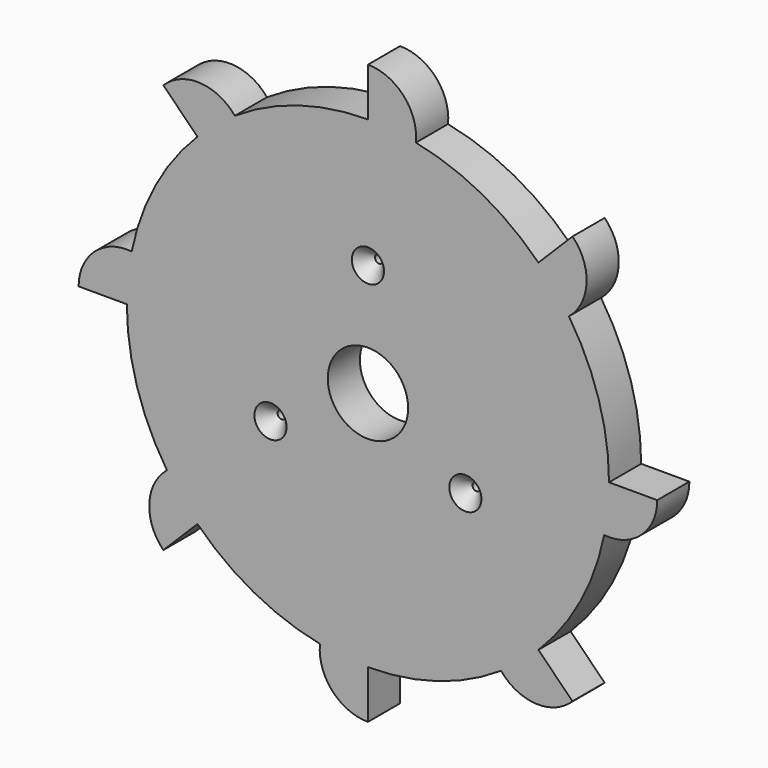
from build123d import *

# Parameters (mm, degrees)
F0_R            = 6.35
F1_DEPTH        = 6.35
F3_D            = 1.27
F3_DEPTH        = 6.35
F3_CSINK_D      = 5.08
F3_CSINK_ANGLE  = 82
F3_TIP          = 0.3815464931
F3_COPIES_COUNT = 3


# Not quite as in the source:
# - a pattern or mirror of a feature is missing from the dataset's text; its kind, count and spacing are read off the source's solid


with BuildPart() as f1:
    # F0 (on Front) → F1 (new body)
    with BuildSketch(Plane.XZ):
        with BuildLine():
            ThreePointArc((37.338, -7.5818042708), (37.9090213538, -3.81), (38.1, 0))
            ThreePointArc((38.1, 0), (36.4813928036, 10.9871733904), (31.7630982094, 21.0408077825))
            ThreePointArc((31.7630982094, 21.0408077825), (29.4998029037, 24.1116492311), (26.9407683632, 26.9407683632))
            ThreePointArc((26.9407683632, 26.9407683632), (18.0271354281, 33.565345049), (7.5818042708, 37.338))
            ThreePointArc((7.5818042708, 37.338), (3.81, 37.9090213538), (0, 38.1))
            ThreePointArc((0, 38.1), (-10.9871733904, 36.4813928036), (-21.0408077825, 31.7630982094))
            ThreePointArc((-21.0408077825, 31.7630982094), (-24.1116492311, 29.4998029037), (-26.9407683632, 26.9407683632))
            ThreePointArc((-26.9407683632, 26.9407683632), (-33.565345049, 18.0271354281), (-37.338, 7.5818042708))
            ThreePointArc((-37.338, 7.5818042708), (-37.9090213538, 3.81), (-38.1, 0))
            ThreePointArc((-38.1, 0), (-36.4813928036, -10.9871733904), (-31.7630982094, -21.0408077825))
            ThreePointArc((-31.7630982094, -21.0408077825), (-29.4998029037, -24.1116492311), (-26.9407683632, -26.9407683632))
            ThreePointArc((-26.9407683632, -26.9407683632), (-18.0271354281, -33.565345049), (-7.5818042708, -37.338))
            ThreePointArc((-7.5818042708, -37.338), (-3.81, -37.9090213538), (0, -38.1))
            ThreePointArc((0, -38.1), (10.9871733904, -36.4813928036), (21.0408077825, -31.7630982094))
            ThreePointArc((21.0408077825, -31.7630982094), (24.1116492311, -29.4998029037), (26.9407683632, -26.9407683632))
            ThreePointArc((26.9407683632, -26.9407683632), (33.565345049, -18.0271354281), (37.338, -7.5818042708))
        make_face()
        Circle(F0_R, mode=Mode.SUBTRACT)
        with BuildLine():
            ThreePointArc((-26.9407683632, 26.9407683632), (-24.1116492311, 29.4998029037), (-21.0408077825, 31.7630982094))
            ThreePointArc((-21.0408077825, 31.7630982094), (-26.5592900173, 34.5512134403), (-32.3289220358, 32.3289220358))
            Line((-32.3289220358, 32.3289220358), (-26.9407683632, 26.9407683632))
        make_face()
        with BuildLine():
            ThreePointArc((0, 38.1), (3.81, 37.9090213538), (7.5818042708, 37.338))
            ThreePointArc((7.5818042708, 37.338), (5.6511432472, 43.2116513966), (0, 45.72))
            Line((0, 45.72), (0, 38.1))
        make_face()
        with BuildLine():
            ThreePointArc((26.9407683632, 26.9407683632), (29.4998029037, 24.1116492311), (31.7630982094, 21.0408077825))
            ThreePointArc((31.7630982094, 21.0408077825), (34.5512134403, 26.5592900173), (32.3289220358, 32.3289220358))
            Line((32.3289220358, 32.3289220358), (26.9407683632, 26.9407683632))
        make_face()
        with BuildLine():
            Line((45.72, 0), (38.1, 0))
            ThreePointArc((38.1, 0), (37.9090213538, -3.81), (37.338, -7.5818042708))
            ThreePointArc((37.338, -7.5818042708), (43.2116513966, -5.6511432472), (45.72, 0))
        make_face()
        with BuildLine():
            Line((32.3289220358, -32.3289220358), (26.9407683632, -26.9407683632))
            ThreePointArc((26.9407683632, -26.9407683632), (24.1116492311, -29.4998029037), (21.0408077825, -31.7630982094))
            ThreePointArc((21.0408077825, -31.7630982094), (26.5592900173, -34.5512134403), (32.3289220358, -32.3289220358))
        make_face()
        with BuildLine():
            Line((0, -45.72), (0, -38.1))
            ThreePointArc((0, -38.1), (-3.81, -37.9090213538), (-7.5818042708, -37.338))
            ThreePointArc((-7.5818042708, -37.338), (-5.6511432472, -43.2116513966), (0, -45.72))
        make_face()
        with BuildLine():
            Line((-32.3289220358, -32.3289220358), (-26.9407683632, -26.9407683632))
            ThreePointArc((-26.9407683632, -26.9407683632), (-29.4998029037, -24.1116492311), (-31.7630982094, -21.0408077825))
            ThreePointArc((-31.7630982094, -21.0408077825), (-34.5512134403, -26.5592900173), (-32.3289220358, -32.3289220358))
        make_face()
        with BuildLine():
            ThreePointArc((-38.1, 0), (-37.9090213538, 3.81), (-37.338, 7.5818042708))
            ThreePointArc((-37.338, 7.5818042708), (-43.2116513966, 5.6511432472), (-45.72, 0))
            Line((-45.72, 0), (-38.1, 0))
        make_face()
    extrude(amount=F1_DEPTH)

    # F3
    with Locations(Plane.XZ.offset(6.35)):
        with Locations((0, 17.78)):
            f3 = CounterSinkHole(F3_D / 2, F3_CSINK_D / 2, depth=F3_DEPTH, counter_sink_angle=F3_CSINK_ANGLE)
            with Locations((0, 0, -(F3_DEPTH + F3_TIP / 2))):  # 118° drill point
                Cone(0, F3_D / 2, F3_TIP, mode=Mode.SUBTRACT)

    # F3_copies: F3 ×3 about axis
    f3_copies_axis = Axis((0, 0, 0), (0, 1, 0))
    for i in range(1, F3_COPIES_COUNT):
        add(f3.rotate(f3_copies_axis, i * 360 / F3_COPIES_COUNT), mode=Mode.SUBTRACT)


solid = f1.part
